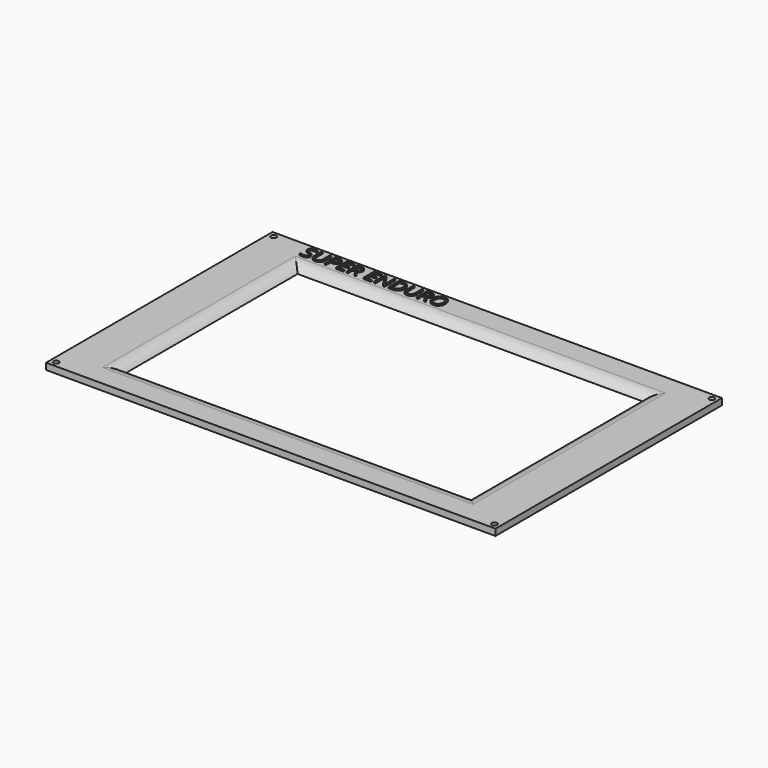
from build123d import *

# Parameters (mm, degrees)
F0_W         = 208
F0_H         = 131
F0_W_2       = 160
F0_H_2       = 100
F1_DEPTH     = 3
F2_T1_DEPTH  = 160
F2_T3_DEPTH  = 100
F2_T9_DEPTH  = 114.3614066163
F2_T13_DEPTH = 174.3614066163
F2_T20_DEPTH = 174.3614066163
F2_T24_DEPTH = 114.3614066163
F2_T31_DEPTH = 174.3614066163
F2_T35_DEPTH = 114.3614066163
F2_T42_DEPTH = 174.3614066163
F2_T46_DEPTH = 114.3614066163
F4_D         = 2.5
F4_DEPTH     = 12
F4_TIP       = 0.7510757738
F5_TEXT_SIZE = 8.8541716751
F6_DEPTH     = 0.5


# Not quite as in the source:
# - a fillet or chamfer that OpenCascade refuses, or shapes differently, is made with other operations: its cross-section is extruded or revolved along the edge and cut away or added
# - Text() gives the source's letters only with a copy of the font that has no kerning and outlines rounded to 1/6400 em; it was checked with that copy


with BuildPart() as f1:
    # F0 (on Top) → F1 (new body)
    with BuildSketch(Plane.XY):
        with Locations((20.5312483013, -8.2446101158)):
            Rectangle(F0_W, F0_H)
        with Locations((20.5312483013, -8.2446101158)):
            Rectangle(F0_W_2, F0_H_2, mode=Mode.SUBTRACT)
    extrude(amount=F1_DEPTH)

    # F2: fillet of radius 7 on 4 edges, made by hand

    # F2_s2 → F2_t1 (cut)
    with BuildSketch(Plane.YZ.offset(-59.4687516987)):
        with BuildLine():
            ThreePointArc((41.7553898842, 0), (44.2595821815, 2.204836823), (47.4999525307, 3))
            Line((47.4999525307, 3), (47.4999525307, 3.14))
            Line((47.4999525307, 3.14), (41.7553898842, 3.14))
            Line((41.7553898842, 3.14), (41.6153898842, 3))
            ThreePointArc((41.6153898842, 3), (41.6153898842, 1.5), (41.6404986312, 0.08))
            Line((41.6404986312, 0.08), (41.7553898842, 0))
        make_face()
        with BuildLine():
            ThreePointArc((-58.2446101158, 0), (-60.7488024132, 2.204836823), (-63.9891727624, 3))
            Line((-63.9891727624, 3), (-63.9891727624, 3.14))
            Line((-63.9891727624, 3.14), (-58.2446101158, 3.14))
            Line((-58.2446101158, 3.14), (-58.1046101158, 3))
            ThreePointArc((-58.1046101158, 3), (-58.1046101158, 1.5), (-58.1297188629, 0.08))
            Line((-58.1297188629, 0.08), (-58.2446101158, 0))
        make_face()
    extrude(amount=F2_T1_DEPTH, mode=Mode.SUBTRACT)

    # F2_s4 → F2_t3 (cut)
    with BuildSketch(Plane.XZ.offset(-41.7553898842)):
        with BuildLine():
            ThreePointArc((-59.4687516987, 0), (-61.9729439961, 2.204836823), (-65.2133143453, 3))
            Line((-65.2133143453, 3), (-65.2133143453, 3.14))
            Line((-65.2133143453, 3.14), (-59.4687516987, 3.14))
            Line((-59.4687516987, 3.14), (-59.3287516987, 3))
            ThreePointArc((-59.3287516987, 3), (-59.3287516987, 1.5), (-59.3538604458, 0.08))
            Line((-59.3538604458, 0.08), (-59.4687516987, 0))
        make_face()
        with BuildLine():
            ThreePointArc((100.5312483013, 0), (103.0354405986, 2.204836823), (106.2758109478, 3))
            Line((106.2758109478, 3), (106.2758109478, 3.14))
            Line((106.2758109478, 3.14), (100.5312483013, 3.14))
            Line((100.5312483013, 3.14), (100.3912483013, 3))
            ThreePointArc((100.3912483013, 3), (100.3912483013, 1.5), (100.4163570483, 0.08))
            Line((100.4163570483, 0.08), (100.5312483013, 0))
        make_face()
    extrude(amount=F2_T3_DEPTH, mode=Mode.SUBTRACT)


with BuildPart() as f2_tool7:
    # F2_s8 → F2_t9 (new body)
    with BuildSketch(Plane.XZ.offset(58.2446101158)):
        with BuildLine():
            ThreePointArc((-59.4687516987, 0), (-61.9729439961, 2.204836823), (-65.2133143453, 3))
            Line((-65.2133143453, 3), (-65.2133143453, 3.14))
            Line((-65.2133143453, 3.14), (-59.4687516987, 3.14))
            Line((-59.4687516987, 3.14), (-59.3287516987, 3))
            ThreePointArc((-59.3287516987, 3), (-59.3287516987, 1.5), (-59.3538604458, 0.08))
            Line((-59.3538604458, 0.08), (-59.4687516987, 0))
        make_face()
    extrude(amount=-F2_T9_DEPTH)

    split(bisect_by=Plane.XZ.offset(-41.7553898842), keep=Keep.BOTTOM)


with BuildPart() as f2_tool11:
    # F2_s12 → F2_t13 (new body)
    with BuildSketch(Plane.YZ.offset(-73.8301583151)):
        with BuildLine():
            ThreePointArc((41.7553898842, 0), (44.2595821815, 2.204836823), (47.4999525307, 3))
            Line((47.4999525307, 3), (47.4999525307, 3.14))
            Line((47.4999525307, 3.14), (41.7553898842, 3.14))
            Line((41.7553898842, 3.14), (41.6153898842, 3))
            ThreePointArc((41.6153898842, 3), (41.6153898842, 1.5), (41.6404986312, 0.08))
            Line((41.6404986312, 0.08), (41.7553898842, 0))
        make_face()
    extrude(amount=F2_T13_DEPTH)

    split(bisect_by=Plane.YZ.offset(-59.4687516987), keep=Keep.BOTTOM)


with BuildPart() as f2_tool7_1:
    add(f2_tool7.part)

    # F2_t15: intersect F2_tool11
    add(f2_tool11.part, mode=Mode.INTERSECT)


with BuildPart() as f1_1:
    add(f1.part)

    # F2_t5: cut F2_tool7
    add(f2_tool7_1.part, mode=Mode.SUBTRACT)


with BuildPart() as f2_tool18:
    # F2_s19 → F2_t20 (new body)
    with BuildSketch(Plane.YZ.offset(-59.4687516987)):
        with BuildLine():
            ThreePointArc((41.7553898842, 0), (44.2595821815, 2.204836823), (47.4999525307, 3))
            Line((47.4999525307, 3), (47.4999525307, 3.14))
            Line((47.4999525307, 3.14), (41.7553898842, 3.14))
            Line((41.7553898842, 3.14), (41.6153898842, 3))
            ThreePointArc((41.6153898842, 3), (41.6153898842, 1.5), (41.6404986312, 0.08))
            Line((41.6404986312, 0.08), (41.7553898842, 0))
        make_face()
    extrude(amount=F2_T20_DEPTH)

    split(bisect_by=Plane.YZ.offset(100.5312483013), keep=Keep.TOP)


with BuildPart() as f2_tool22:
    # F2_s23 → F2_t24 (new body)
    with BuildSketch(Plane.XZ.offset(-56.1167965005)):
        with BuildLine():
            ThreePointArc((100.5312483013, 0), (103.0354405986, 2.204836823), (106.2758109478, 3))
            Line((106.2758109478, 3), (106.2758109478, 3.14))
            Line((106.2758109478, 3.14), (100.5312483013, 3.14))
            Line((100.5312483013, 3.14), (100.3912483013, 3))
            ThreePointArc((100.3912483013, 3), (100.3912483013, 1.5), (100.4163570483, 0.08))
            Line((100.4163570483, 0.08), (100.5312483013, 0))
        make_face()
    extrude(amount=F2_T24_DEPTH)

    split(bisect_by=Plane.XZ.offset(-41.7553898842), keep=Keep.BOTTOM)


with BuildPart() as f2_tool18_1:
    add(f2_tool18.part)

    # F2_t26: intersect F2_tool22
    add(f2_tool22.part, mode=Mode.INTERSECT)


with BuildPart() as f1_2:
    add(f1_1.part)

    # F2_t16: cut F2_tool18
    add(f2_tool18_1.part, mode=Mode.SUBTRACT)


with BuildPart() as f2_tool29:
    # F2_s30 → F2_t31 (new body)
    with BuildSketch(Plane.YZ.offset(100.5312483013)):
        with BuildLine():
            ThreePointArc((-58.2446101158, 0), (-60.7488024132, 2.204836823), (-63.9891727624, 3))
            Line((-63.9891727624, 3), (-63.9891727624, 3.14))
            Line((-63.9891727624, 3.14), (-58.2446101158, 3.14))
            Line((-58.2446101158, 3.14), (-58.1046101158, 3))
            ThreePointArc((-58.1046101158, 3), (-58.1046101158, 1.5), (-58.1297188629, 0.08))
            Line((-58.1297188629, 0.08), (-58.2446101158, 0))
        make_face()
    extrude(amount=-F2_T31_DEPTH)

    split(bisect_by=Plane.YZ.offset(-59.4687516987), keep=Keep.BOTTOM)


with BuildPart() as f2_tool33:
    # F2_s34 → F2_t35 (new body)
    with BuildSketch(Plane.XZ.offset(72.6060167322)):
        with BuildLine():
            ThreePointArc((-59.4687516987, 0), (-61.9729439961, 2.204836823), (-65.2133143453, 3))
            Line((-65.2133143453, 3), (-65.2133143453, 3.14))
            Line((-65.2133143453, 3.14), (-59.4687516987, 3.14))
            Line((-59.4687516987, 3.14), (-59.3287516987, 3))
            ThreePointArc((-59.3287516987, 3), (-59.3287516987, 1.5), (-59.3538604458, 0.08))
            Line((-59.3538604458, 0.08), (-59.4687516987, 0))
        make_face()
    extrude(amount=-F2_T35_DEPTH)

    split(bisect_by=Plane.XZ.offset(58.2446101158), keep=Keep.TOP)


with BuildPart() as f2_tool29_1:
    add(f2_tool29.part)

    # F2_t37: intersect F2_tool33
    add(f2_tool33.part, mode=Mode.INTERSECT)


with BuildPart() as f1_3:
    add(f1_2.part)

    # F2_t27: cut F2_tool29
    add(f2_tool29_1.part, mode=Mode.SUBTRACT)


with BuildPart() as f2_tool40:
    # F2_s41 → F2_t42 (new body)
    with BuildSketch(Plane.YZ.offset(114.8926549176)):
        with BuildLine():
            ThreePointArc((-58.2446101158, 0), (-60.7488024132, 2.204836823), (-63.9891727624, 3))
            Line((-63.9891727624, 3), (-63.9891727624, 3.14))
            Line((-63.9891727624, 3.14), (-58.2446101158, 3.14))
            Line((-58.2446101158, 3.14), (-58.1046101158, 3))
            ThreePointArc((-58.1046101158, 3), (-58.1046101158, 1.5), (-58.1297188629, 0.08))
            Line((-58.1297188629, 0.08), (-58.2446101158, 0))
        make_face()
    extrude(amount=-F2_T42_DEPTH)

    split(bisect_by=Plane.YZ.offset(100.5312483013), keep=Keep.TOP)


with BuildPart() as f2_tool44:
    # F2_s45 → F2_t46 (new body)
    with BuildSketch(Plane.XZ.offset(-41.7553898842)):
        with BuildLine():
            ThreePointArc((100.5312483013, 0), (103.0354405986, 2.204836823), (106.2758109478, 3))
            Line((106.2758109478, 3), (106.2758109478, 3.14))
            Line((106.2758109478, 3.14), (100.5312483013, 3.14))
            Line((100.5312483013, 3.14), (100.3912483013, 3))
            ThreePointArc((100.3912483013, 3), (100.3912483013, 1.5), (100.4163570483, 0.08))
            Line((100.4163570483, 0.08), (100.5312483013, 0))
        make_face()
    extrude(amount=F2_T46_DEPTH)

    split(bisect_by=Plane.XZ.offset(58.2446101158), keep=Keep.TOP)


with BuildPart() as f2_tool40_1:
    add(f2_tool40.part)

    # F2_t48: intersect F2_tool44
    add(f2_tool44.part, mode=Mode.INTERSECT)


with BuildPart() as f1_4:
    add(f1_3.part)

    # F2_t38: cut F2_tool40
    add(f2_tool40_1.part, mode=Mode.SUBTRACT)

    # F4
    with Locations(Plane.XY.offset(3)):
        with Locations((-80.8687516987, 54.6553898842), (121.9312483013, 54.6553898842), (121.9312483013, -71.1446101158), (-80.8687516987, -71.1446101158)):
            Hole(F4_D / 2, depth=F4_DEPTH)
            with Locations((0, 0, -(F4_DEPTH + F4_TIP / 2))):  # 118° drill point
                Cone(0, F4_D / 2, F4_TIP, mode=Mode.SUBTRACT)

    # F5 (on face) → F6 (join)
    with BuildSketch(Plane.XY.offset(3)):
        with Locations((-65.0625005364, 49.0312501788)):
            Text('SUPER ENDURO', F5_TEXT_SIZE, font='Open Sans', text_align=(TextAlign.LEFT, TextAlign.BOTTOM))
    extrude(amount=F6_DEPTH)


solid = f1_4.part
